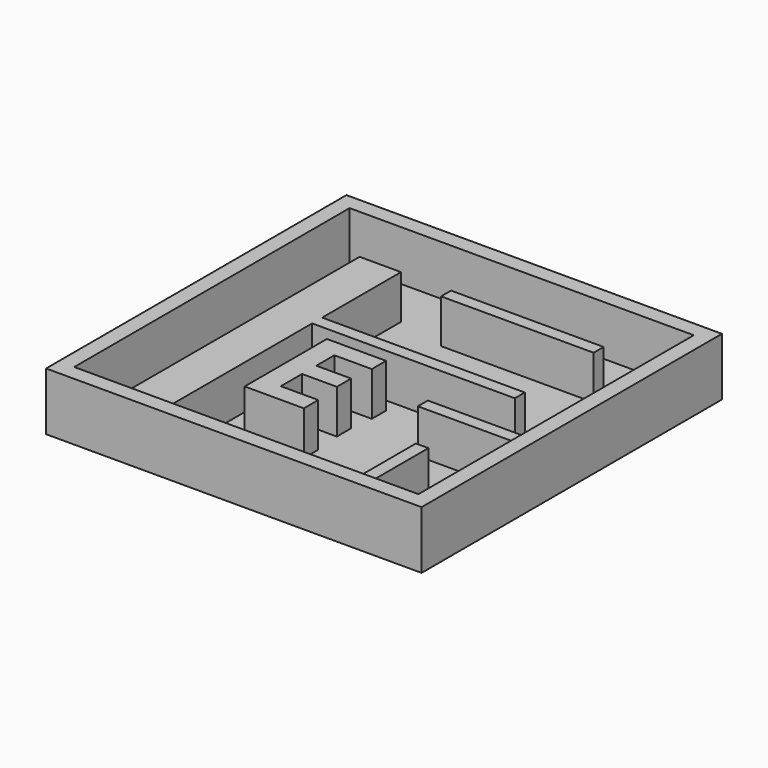
from build123d import *

# Parameters (mm, degrees)
F0_W         = 38.1
F0_H         = 38.1
F1_DEPTH     = 0.79375
F2_W         = 38.1
F2_H         = 38.1
F2_W_2       = 34.925
F2_H_2       = 34.925
F3_DEPTH     = 5.08
F4_TEXT_SIZE = 14.6134568947
F4_W         = 15.4837645781
F4_H         = 1.27
F4_W_2       = 10.2202369381
F4_W_3       = 1.27
F4_H_2       = 7.62
F5_DEPTH     = 4.445


# Not quite as in the source:
# - Text() gives the source's letters only with a copy of the font that has no kerning and outlines rounded to 1/6400 em; it was checked with that copy


with BuildPart() as f1:
    # F0 (on Top) → F1 (new body)
    with BuildSketch(Plane.XY):
        with Locations((-3.701062873, -0.5359856714)):
            Rectangle(F0_W, F0_H)
    extrude(amount=F1_DEPTH)

    # F2 (on face) → F3 (join)
    with BuildSketch(Plane.XY.offset(0.79375)):
        with Locations((-3.701062873, -0.5359856714)):
            Rectangle(F2_W, F2_H)
        with Locations((-3.701062873, -0.5359856714)):
            Rectangle(F2_W_2, F2_H_2, mode=Mode.SUBTRACT)
    extrude(amount=F3_DEPTH)

    # F4 (on face) → F5 (join)
    with BuildSketch(Plane.XY.offset(0.79375)):
        with Locations((-10.6123274511, -11.2150934285)):
            Text('E', F4_TEXT_SIZE, font='Open Sans', font_style=FontStyle.BOLD, text_align=(TextAlign.LEFT, TextAlign.BOTTOM))
        Polygon((-16.083562873, 11.8465143286), (-16.083562873, -17.9984856714), (-11.8823274511, -17.9984856714), (-11.8823274511, 0.5765955357), (8.681437127, 0.5765955357), (8.681437127, 1.8465955357), (-11.8823274511, 1.8465955357), (-11.8823274511, 11.8465143286), align=None)
        with Locations((0.939554838, 11.2115143286)):
            Rectangle(F4_W, F4_H)
        with Locations((8.651318658, -4.6634856714)):
            Rectangle(F4_W_2, F4_H)
        with Locations((8.046437127, -14.1884856714)):
            Rectangle(F4_W_3, F4_H_2)
    extrude(amount=F5_DEPTH)


solid = f1.part
